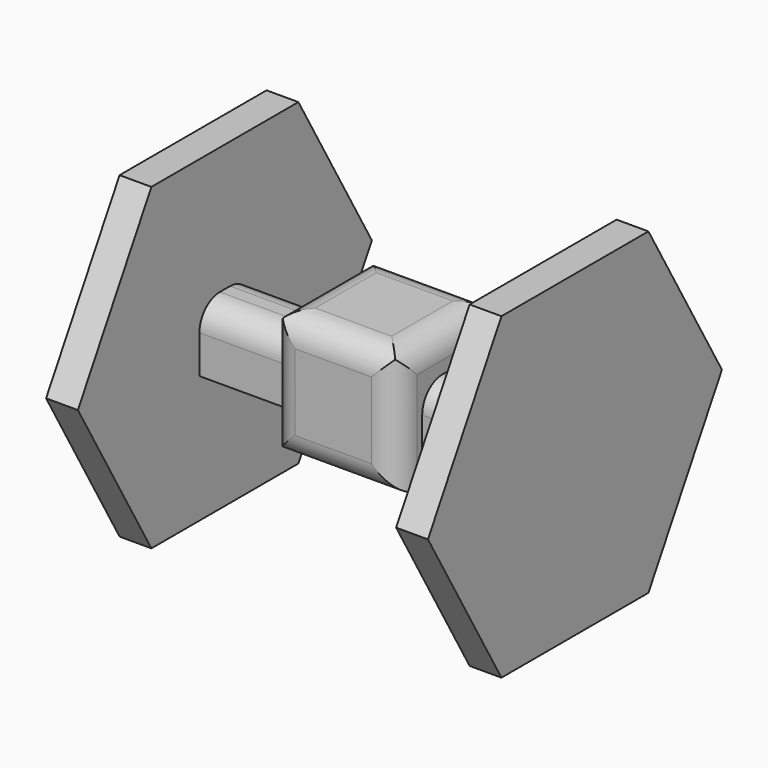
from build123d import *

# Parameters (mm, degrees)
F0_W         = 12.7
F0_H         = 12.7
F1_DEPTH     = 38.1
F2_R         = 5.08
F3_W         = 25.4
F3_H         = 25.4
F4_DEPTH     = 12.7
F6_DEPTH     = 6.35
F8_R         = 5.08
F9_T1_DEPTH  = 45.72
F9_T3_DEPTH  = 50.8
F10_T1_DEPTH = 45.72
F10_T3_DEPTH = 50.8


# Not quite as in the source:
# - a fillet or chamfer that OpenCascade refuses, or shapes differently, is made with other operations: its cross-section is extruded or revolved along the edge and cut away or added


with BuildPart() as f1:
    # F0 (on Right) → F1 (new body)
    with BuildSketch(Plane.YZ):
        Rectangle(F0_W, F0_H)
    extrude(amount=F1_DEPTH)

    # F2
    f2_edges = [f1.edges().sort_by_distance(p)[0] for p in [
        (19.05, 6.35, 6.35),
        (19.05, -6.35, 6.35),
        (0, 0, 6.35),
    ]]
    fillet(f2_edges, radius=F2_R)

    # F3 (on Right) → F4 (join)
    with BuildSketch(Plane.YZ):
        with Locations((0, 1.27)):
            Rectangle(F3_W, F3_H)
    extrude(amount=F4_DEPTH)

    # F5 (on face) → F6 (join)
    with BuildSketch(Plane.YZ.offset(38.1)):
        Polygon((-18.3308710468, -31.75), (18.3308710468, -31.75), (36.6617420935, 0), (18.3308710468, 31.75), (-18.3308710468, 31.75), (-36.6617420935, 0), align=None)
    extrude(amount=-F6_DEPTH)

    # F7: F1 across plane


with BuildPart() as f1_1:
    add(f1.part)
    add(f1.part.mirror(Plane.YZ))

    # F8
    f8_edges = [f1_1.edges().sort_by_distance(p)[0] for p in [
        (12.7, 0, 13.97),
        (0, -12.7, 13.97),
        (-12.7, 0, 13.97),
        (0, 12.7, 13.97),
    ]]
    fillet(f8_edges, radius=F8_R)

    # F9: fillet of radius 5.08 on 4 edges, made by hand

    # F9_s2 → F9_t1 (cut)
    with BuildSketch(Plane.XY.offset(-24.13)):
        with BuildLine():
            ThreePointArc((12.7, -7.62), (11.2121024484, -11.2121024484), (7.62, -12.7))
            Line((7.62, -12.7), (12.7, -12.7))
            Line((12.7, -12.7), (12.7, -7.62))
        make_face()
        with BuildLine():
            ThreePointArc((-7.62, -12.7), (-11.2121024484, -11.2121024484), (-12.7, -7.62))
            Line((-12.7, -7.62), (-12.7, -12.7))
            Line((-12.7, -12.7), (-7.62, -12.7))
        make_face()
    extrude(amount=F9_T1_DEPTH, mode=Mode.SUBTRACT)

    # F9_s4 → F9_t3 (cut)
    with BuildSketch(Plane.YZ.offset(-25.4)):
        with BuildLine():
            ThreePointArc((-7.62, -11.43), (-11.2121024484, -9.9421024484), (-12.7, -6.35))
            Line((-12.7, -6.35), (-12.7, -11.43))
            Line((-12.7, -11.43), (-7.62, -11.43))
        make_face()
    extrude(amount=F9_T3_DEPTH, mode=Mode.SUBTRACT)

    # F10: fillet of radius 5.08 on 4 edges, made by hand

    # F10_s2 → F10_t1 (cut)
    with BuildSketch(Plane.XY.offset(-24.13)):
        with BuildLine():
            ThreePointArc((12.7, 7.62), (11.2121024484, 11.2121024484), (7.62, 12.7))
            Line((7.62, 12.7), (12.7, 12.7))
            Line((12.7, 12.7), (12.7, 7.62))
        make_face()
        with BuildLine():
            ThreePointArc((-7.62, 12.7), (-11.2121024484, 11.2121024484), (-12.7, 7.62))
            Line((-12.7, 7.62), (-12.7, 12.7))
            Line((-12.7, 12.7), (-7.62, 12.7))
        make_face()
    extrude(amount=F10_T1_DEPTH, mode=Mode.SUBTRACT)

    # F10_s4 → F10_t3 (cut)
    with BuildSketch(Plane.YZ.offset(-25.4)):
        with BuildLine():
            ThreePointArc((12.7, -6.35), (11.2121024484, -9.9421024484), (7.62, -11.43))
            Line((7.62, -11.43), (12.7, -11.43))
            Line((12.7, -11.43), (12.7, -6.35))
        make_face()
    extrude(amount=F10_T3_DEPTH, mode=Mode.SUBTRACT)


solid = f1_1.part
